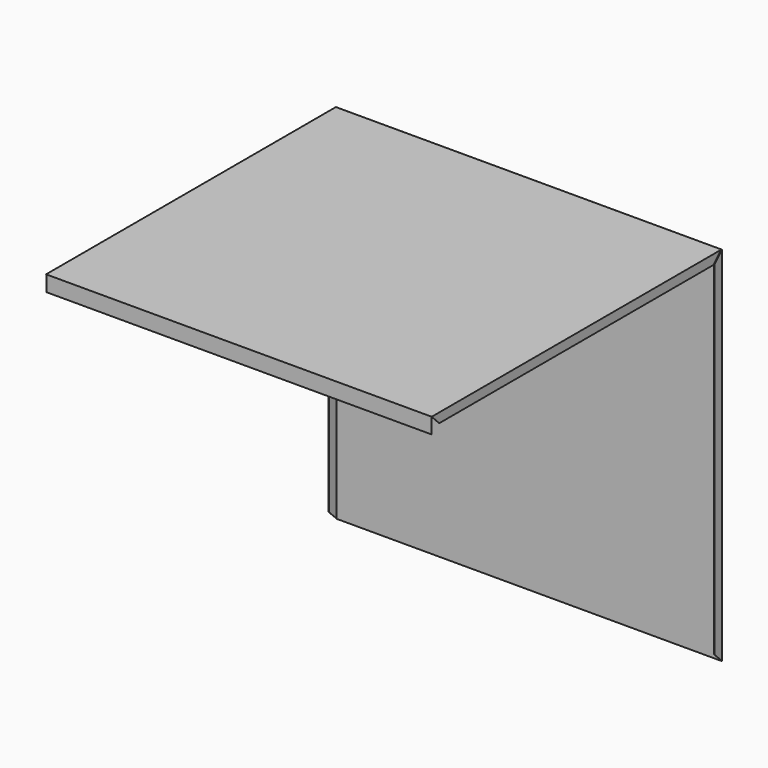
from build123d import *

# Parameters (mm, degrees)
F1_DEPTH = 641.35
F2_R     = 2.54
F4_DEPTH = 1.27


# Not quite as in the source:
# - a pattern or mirror of a feature is missing from the dataset's text; its kind, count and spacing are read off the source's solid


with BuildPart() as f1:
    # F0 (on Right) → F1 (new body, symmetric)
    with BuildSketch(Plane.YZ):
        Polygon((-1.27, 0), (0, 0), (0, 50.8), (1206.5, 50.8), (1206.5, -1155.7), (1207.77, -1155.7), (1207.77, 52.07), (-1.27, 52.07), align=None)
    extrude(amount=F1_DEPTH, both=True)

    # F2
    f2_edges = [f1.edges().sort_by_distance(p)[0] for p in [
        (0, 1207.77, 52.07),
    ]]
    fillet(f2_edges, radius=F2_R)

    # F3 (on face) → F4 (join)
    with BuildSketch(Plane.YZ.offset(641.35)):
        with BuildLine():
            Line((1205.23, 52.07), (-1.27, 52.07))
            Line((-1.27, 52.07), (30.48, 20.32))
            Line((30.48, 20.32), (1172.2684317215, 20.32))
            Line((1172.2684317215, 20.32), (1204.2542837185, 50.8))
            Line((1204.2542837185, 50.8), (1206.5, 50.8))
            Line((1206.5, 50.8), (1206.5, 48.5542837185))
            Line((1206.5, 48.5542837185), (1176.02, 19.5092421769))
            Line((1176.02, 19.5092421769), (1176.02, -1123.95))
            Line((1176.02, -1123.95), (1207.77, -1155.7))
            Line((1207.77, -1155.7), (1207.77, -1123.95))
            Line((1207.77, -1123.95), (1207.77, 49.53))
            ThreePointArc((1207.77, 49.53), (1207.0260512242, 51.3260512242), (1205.23, 52.07))
        make_face()
    f4 = extrude(amount=F4_DEPTH)

    # F4_copies: F4 across plane
    add(f4.mirror(Plane(origin=(0, 0, 0), x_dir=(0, 0, -1), z_dir=(-1, 0, 0))))


solid = f1.part
